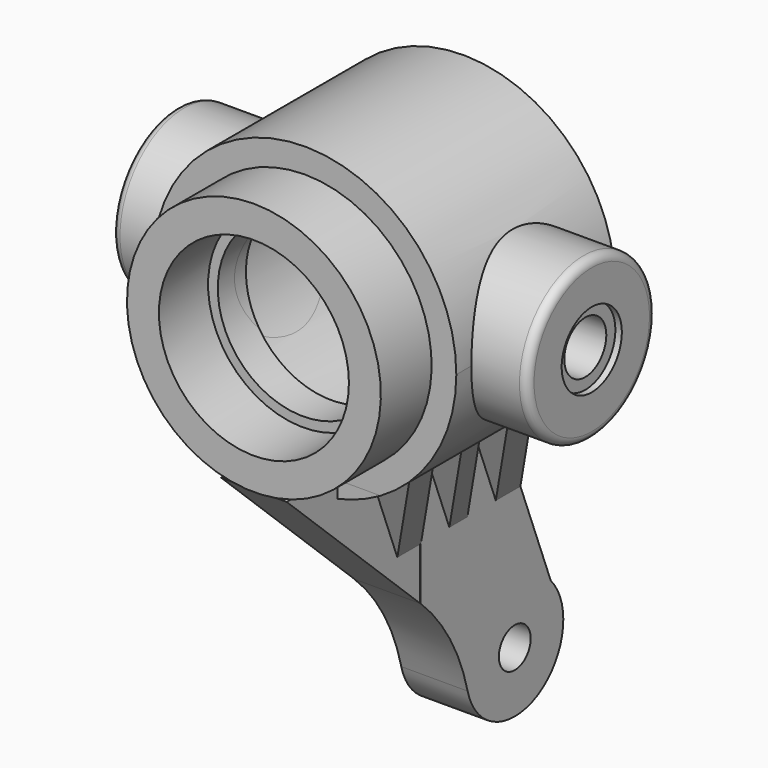
from build123d import *

# Parameters (mm, degrees)
F0_R      = 9.525
F0_R_2    = 5.3594
F1_DEPTH  = 16.4338
F2_R      = 7.4549
F2_R_2    = 5.3594
F3_DEPTH  = 10.3632
F4_R      = 5.969
F5_DEPTH  = 3.8608
F6_R      = 9.525
F6_R_2    = 7.9756
F7_DEPTH  = 3.9878
F8_R      = 5.0419
F9_DEPTH  = 13.0556
F14_DEPTH = 2.0574
F16_DEPTH = 2.0828
F18_D     = 2.5
F19_R     = 0.508
F20_R     = 2.3622
F21_DEPTH = 0.4064
F25_DEPTH = 14.3256
F27_DEPTH = 12.7
F29_DEPTH = 25.4
F31_DEPTH = 12.446
F32_R     = 1.64973
F33_DEPTH = 5.4864


# Not quite as in the source:
# - a pattern or mirror of a feature is missing from the dataset's text; its kind, count and spacing are read off the source's solid


with BuildPart() as f1:
    # F0 (on Front) → F1 (new body)
    with BuildSketch(Plane.XZ):
        Circle(F0_R)
        Circle(F0_R_2, mode=Mode.SUBTRACT)
    extrude(amount=F1_DEPTH)

    # F2 (on face) → F3 (cut)
    with BuildSketch(Plane(origin=(0, 0, 0), x_dir=(-1, 0, 0), z_dir=(0, 1, 0))):
        Circle(F2_R)
        Circle(F2_R_2, mode=Mode.SUBTRACT)
    extrude(amount=-F3_DEPTH, mode=Mode.SUBTRACT)

    # F4 (on face) → F5 (cut)
    with BuildSketch(Plane.XZ.offset(16.4338)):
        Circle(F4_R)
    extrude(amount=-F5_DEPTH, mode=Mode.SUBTRACT)

    # F6 (on face) → F7 (cut)
    with BuildSketch(Plane.XZ.offset(16.4338)):
        Circle(F6_R)
        Circle(F6_R_2, mode=Mode.SUBTRACT)
    extrude(amount=-F7_DEPTH, mode=Mode.SUBTRACT)

    # F8 (on Right) → F9 (join, symmetric)
    with BuildSketch(Plane.YZ):
        with Locations((-6.223, 0)):
            Circle(F8_R)
    extrude(amount=F9_DEPTH, both=True)

    # F11 (on Top) → F12 (revolve, cut)
    with BuildSketch(Plane.XY):
        Polygon((0, 0), (-7.4549, 0), (-7.4549, -10.3632), (-5.3594, -10.3632), (-5.3594, -10.368520394), (-5.3594, -12.573), (-5.969, -12.573), (-5.969, -16.4338), (0, -16.4338), align=None)
    revolve(axis=Axis((0, -8.2169, 0), (0, -1, 0)), mode=Mode.SUBTRACT)

    # F13 (on Right) → F14 (join, symmetric)
    with BuildSketch(Plane.YZ):
        Polygon((-5.9436, -7.8486), (-16.4338, -7.8486), (-5.9436, -17.7292), align=None)
    extrude(amount=F14_DEPTH, both=True)

    # F15 (on Right) → F16 (join, symmetric)
    with BuildSketch(Plane.YZ):
        with BuildLine():
            ThreePointArc((-5.9436, -17.7292), (-3.63902226, -20.6305545993), (-2.2538056534, -24.0671389535))
            ThreePointArc((-2.2538056534, -24.0671389535), (3.2323921711, -26.5310042099), (4.2720160752, -20.607476485))
            Line((4.2720160752, -20.607476485), (0, -9.525))
            Line((0, -9.525), (0, -8.255))
            Line((0, -8.255), (-5.9436, -8.255))
            Line((-5.9436, -8.255), (-5.9436, -9.525))
            Line((-5.9436, -9.525), (-5.9436, -17.7292))
        make_face()
    extrude(amount=F16_DEPTH, both=True)

    # F18 (through all)
    with Locations(Plane.YZ.offset(2.0828)):
        with Locations((1.4478, -23.1648)):
            Hole(F18_D / 2)

    # F19
    f19_edges = [f1.edges().sort_by_distance(p)[0] for p in [
        (13.0556, -11.2649, 0),
        (-13.0556, -11.2649, 0),
    ]]
    fillet(f19_edges, radius=F19_R)

    # F20 (on face) → F21 (cut)
    with BuildSketch(Plane.YZ.offset(13.0556)):
        with Locations((-6.223, 0)):
            Circle(F20_R)
    f21 = extrude(amount=-F21_DEPTH, mode=Mode.SUBTRACT)

    # F21_copies: F21 across plane
    add(f21.mirror(Plane(origin=(0, 0, 0), x_dir=(0, 0, -1), z_dir=(-1, 0, 0))), mode=Mode.SUBTRACT)

    # F24 (on plane+point) → F25 (join)
    with BuildSketch(Plane.XZ.offset(-1.8896748603)):
        Polygon((2.0828, -8.248891971), (2.0828, -14.4272), (4.7625, -8.248891971), align=None)
    f25 = extrude(amount=F25_DEPTH)

    # F25_copies: F25 across plane
    add(f25.mirror(Plane(origin=(0, 0, 0), x_dir=(0, 0, -1), z_dir=(-1, 0, 0))))

    # F26 (on face) → F27 (cut, symmetric)
    with BuildSketch(Plane.YZ.offset(2.0828)):
        Polygon((0, -8.248891971), (0, -9.525), (1.8896748603, -14.4272), (1.8896748603, -8.248891971), align=None)
    extrude(amount=F27_DEPTH, both=True, mode=Mode.SUBTRACT)

    # F28 (on face) → F29 (cut)
    with BuildSketch(Plane.YZ.offset(2.0828)):
        Polygon((-2.2752562937, -14.4272), (-0.0430709693, -14.4272), (-2.4246533939, -8.248891971), (-4.6568387183, -8.248891971), align=None)
        Polygon((-5.9229737751, -14.4272), (-3.6907884507, -14.4272), (-6.0723708752, -8.248891971), (-8.3045561996, -8.248891971), align=None)
        Polygon((-12.4359251397, -14.4272), (-7.774054288, -14.4272), (-10.1556367126, -8.248891971), (-12.4359251397, -8.248891971), align=None)
    f29 = extrude(amount=F29_DEPTH, mode=Mode.SUBTRACT)

    # F29_copies: F29 across plane
    add(f29.mirror(Plane(origin=(0, 0, 0), x_dir=(0, 0, -1), z_dir=(-1, 0, 0))), mode=Mode.SUBTRACT)

    # F30 (on face) → F31 (join, through all)
    with BuildSketch(Plane.XZ.offset(12.446)):
        with BuildLine():
            Line((2.0828, -8.248891971), (-4.7625, -8.248891971))
            ThreePointArc((-4.7625, -8.248891971), (0, -9.525), (4.7625, -8.248891971))
            Line((4.7625, -8.248891971), (2.0828, -8.248891971))
        make_face()
    extrude(amount=-F31_DEPTH)

    # F32 (on face) → F33 (cut)
    with BuildSketch(Plane.YZ.offset(13.0556)):
        with Locations((-6.223, 0)):
            Circle(F32_R)
    f33 = extrude(amount=-F33_DEPTH, mode=Mode.SUBTRACT)

    # F33_copies: F33 across plane
    add(f33.mirror(Plane(origin=(0, 0, 0), x_dir=(0, 0, -1), z_dir=(-1, 0, 0))), mode=Mode.SUBTRACT)


solid = f1.part
